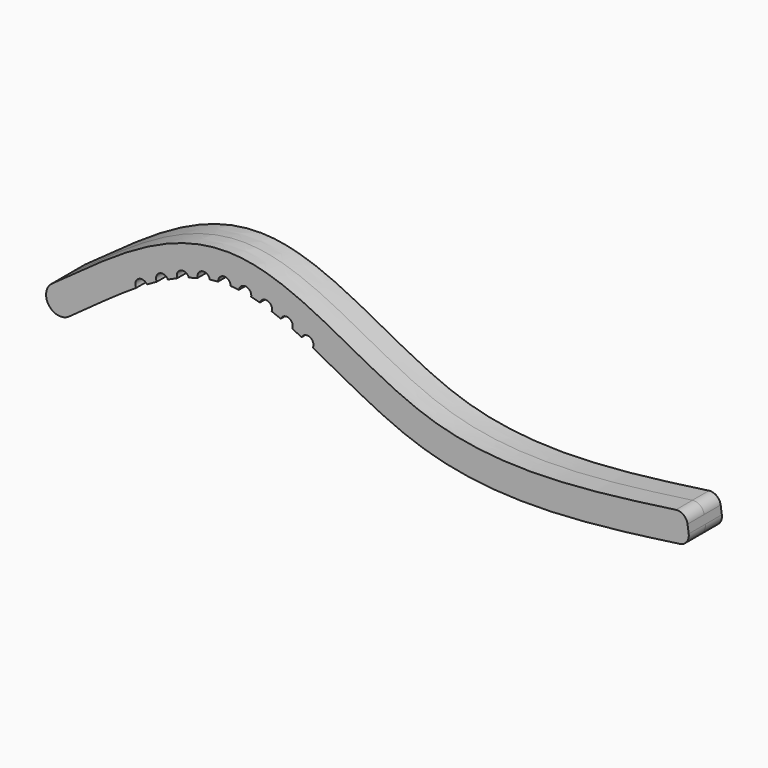
from build123d import *

# Parameters (mm, degrees)
F1_DEPTH = 5
F2_R     = 2.5
F3_R     = 1.5
F4_DEPTH = 10.0010001


# Not quite as in the source:
# - the dataset's text gives a spline's control points without its knots; the knots are read off the source's solid


with BuildPart() as f1:
    # F0 (on Front) → F1 (new body, symmetric)
    with BuildSketch(Plane.XZ):
        with BuildLine():
            ThreePointArc((-4.0449113911, 5.7130282546), (-4.8789698229, 0.8340584318), (0, 0))
            add(Edge.make_bspline(
                [(0, 0), (12.6866183221, 8.9823198273), (39.097046681, 31.0254585121), (84.6231120805, -9.3204370609), (127.451649596, -3.1579744512), (150, 0)],
                knots=[0, 0, 0, 0, 0.3024009423, 0.6287352131, 1, 1, 1, 1], degree=3))
            Line((150, 0), (149.0291016229, 6.9323413319))
            add(Edge.make_bspline(
                [(-4.0449113911, 5.7130282546), (-1.4893265055, 7.522421444), (2.4289578755, 10.3991251109), (7.8311540893, 14.2258677584), (11.985518828, 17.0073967049), (16.2624014486, 19.6143417246), (20.6904437749, 21.9553087459), (25.3048430013, 23.9276125636), (29.3354802395, 25.1619067391), (32.6783528938, 25.828942319), (35.2427144442, 26.1479585874), (37.419626365, 26.2456905562), (39.1857443489, 26.2125714545), (40.9384858731, 26.1049312213), (43.0954900321, 25.8409787708), (46.4720299209, 25.1788075072), (50.5545204313, 23.9683165065), (55.2777949463, 22.0808731164), (59.8806691618, 19.8983979978), (64.4079741748, 17.5399643684), (68.8916038218, 15.1143270568), (73.3515183232, 12.7253635973), (77.7977758185, 10.4736185968), (81.4936492304, 8.7918611912), (84.4432333572, 7.608120023), (86.2840306834, 6.9438576049), (87.7535671011, 6.4632867232), (89.2383433444, 6.0114309597), (91.1197744412, 5.5000916427), (93.4192059549, 4.9686735981), (96.5398637001, 4.3656966777), (100.5419436116, 3.8023805188), (105.4978361754, 3.4066907033), (110.5952082283, 3.2657358671), (117.5618909593, 3.3809979789), (126.5522503494, 4.0218977706), (137.6717582852, 5.3370647038), (145.2302773967, 6.4003028618), (149.0291016229, 6.9323413319)],
                knots=[0, 0, 0, 0, 0.0625, 0.09375, 0.125, 0.15625, 0.1875, 0.21875, 0.25, 0.265625, 0.28125, 0.296875, 0.3046875, 0.3125, 0.328125, 0.34375, 0.375, 0.40625, 0.4375, 0.46875, 0.5, 0.53125, 0.5625, 0.59375, 0.609375, 0.625, 0.6328125, 0.640625, 0.65625, 0.671875, 0.6875, 0.71875, 0.75, 0.78125, 0.8125, 0.875, 0.9375, 1, 1, 1, 1], degree=3))
        make_face()
    extrude(amount=F1_DEPTH, both=True)

    # F2
    f2_edges = [f1.edges().sort_by_distance(p)[0] for p in [
        (149.029102, 2.5, 6.932341),
        (150, 2.5, 0),
        (149.029102, -2.5, 6.932341),
        (150, -2.5, 0),
    ]]
    fillet(f2_edges, radius=F2_R)

    # F3 (on face) → F4 (cut, through all)
    with BuildSketch(Plane.XZ.offset(5)):
        with Locations((37.5310791936, 19.2248344713)):
            Circle(F3_R)
        with Locations((32.5310791936, 18.6530319414)):
            Circle(F3_R)
        with Locations((27.5310791936, 17.192316528)):
            Circle(F3_R)
        with Locations((22.5310791936, 14.983407983)):
            Circle(F3_R)
        with Locations((17.5310791936, 12.1773542976)):
            Circle(F3_R)
        with Locations((42.5310791936, 18.806197108)):
            Circle(F3_R)
        with Locations((47.5310791936, 17.51930095)):
            Circle(F3_R)
        with Locations((52.5310791936, 15.5840389676)):
            Circle(F3_R)
        with Locations((57.5310791936, 13.2102312001)):
            Circle(F3_R)
    extrude(amount=-F4_DEPTH, mode=Mode.SUBTRACT)


solid = f1.part
